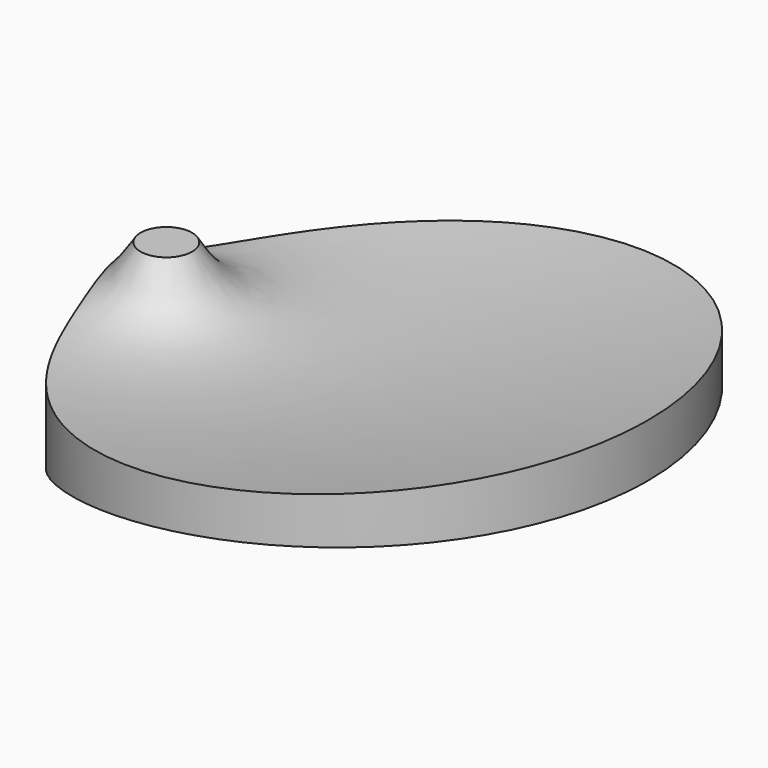
from build123d import *

# Parameters (mm, degrees)
F4_START = -150
F0_R     = 200
F4_DEPTH = 180


with BuildPart() as f3:
    # F2 (on Front) → F3 (revolve)
    with BuildSketch(Plane.XZ):
        with BuildLine():
            Line((0, -150), (19.5, -150))
            add(Edge.make_bspline(
                [(19.5, -150), (59.0057506558, -66.050296319), (248.9092350006, -23.7886533141), (365, -10.3441393003)],
                knots=[0, 0, 0, 0, 372.6580328234, 372.6580328234, 372.6580328234, 372.6580328234], degree=3))
            Line((365, -10.3441393003), (365, 30))
            add(Edge.make_bspline(
                [(19.5, 30), (27.6682462512, 17.1148710825), (53.7917624642, -33.3818905483), (261.0534458626, 3.9776707628), (365, 30)],
                knots=[0, 0, 0, 0, 0.2911930503, 1, 1, 1, 1], degree=3))
            Line((19.5, 30), (0, 30))
            Line((0, 30), (0, -150))
        make_face()
    revolve(axis=Axis((0, 0, -60), (0, 0, -1)))

    # F0 (on Top) → F4 (intersect)
    with BuildSketch(Plane.XY.offset(F4_START)):
        with Locations((165, 0)):
            Circle(F0_R)
    extrude(amount=F4_DEPTH, mode=Mode.INTERSECT)


solid = f3.part
